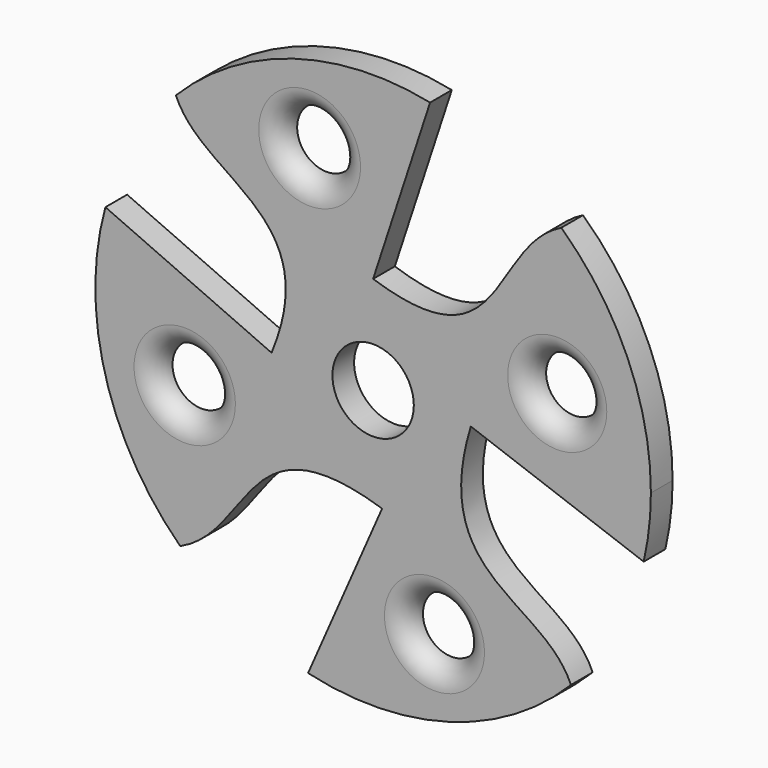
from build123d import *

# Parameters (mm, degrees)
F0_R     = 12.5871716163
F0_R_2   = 12.1953483152
F0_R_3   = 12.6822409032
F0_R_4   = 19.9906816782
F0_R_5   = 12.6370181024
F0_R_6   = 9.5235294205
F0_R_7   = 6.7003849176
F0_R_8   = 6.5953683563
F0_R_9   = 6.9128696082
F0_R_10  = 6.8565575186
F1_DEPTH = 6.35
F2_R     = 5
F4_R     = 5
F6_R     = 5
F8_R     = 5


# Not quite as in the source:
# - a fillet or chamfer that OpenCascade refuses, or shapes differently, is made with other operations: its cross-section is extruded or revolved along the edge and cut away or added


with BuildPart() as f1:
    # F0 (on Front) → F1 (new body)
    with BuildSketch(Plane.XZ):
        with BuildLine():
            ThreePointArc((63.3090875557, -14.7056564815), (64.571840502, -7.4009670899), (64.994591311, 0))
            ThreePointArc((64.994591311, 0), (59.5228001423, 26.1023593361), (44.0287494104, 47.8096865189))
            add(Edge.make_bspline(
                [(44.0287494104, 47.8096865189), (27.5113759255, 39.6058435289), (31.2073216603, 12.5460234383), (0, 22.9526739568)],
                knots=[0, 0, 0, 0, 50.5608726998, 50.5608726998, 50.5608726998, 50.5608726998], degree=3))
            Line((0, 22.9526739568), (13.3303934836, 63.6128721978))
            ThreePointArc((13.3303934836, 63.6128721978), (-18.6797347685, 62.2524249219), (-46.1507096662, 45.7647123556))
            add(Edge.make_bspline(
                [(-46.1507096662, 45.7647123556), (-39.6496795631, 30.4512329053), (-10.8062981221, 31.6188670695), (-23.7553194165, 0)],
                knots=[0, 0, 0, 0, 50.9505878418, 50.9505878418, 50.9505878418, 50.9505878418], degree=3))
            Line((-23.7553194165, 0), (-62.6320905617, 17.3642774556))
            ThreePointArc((-62.6320905617, 17.3642774556), (-62.7024955301, -17.1083007333), (-45.133666011, -46.7680349394))
            add(Edge.make_bspline(
                [(-45.133666011, -46.7680349394), (-28.2305709499, -39.1496551166), (-30.3561454639, -13.2581368089), (2.106344793, -23.6651096493)],
                knots=[0, 0, 0, 0, 52.5867262502, 52.5867262502, 52.5867262502, 52.5867262502], degree=3))
            Line((2.106344793, -23.6651096493), (-15.2139644468, -63.1888612454))
            ThreePointArc((-15.2139644468, -63.1888612454), (17.847761713, -62.4960342863), (46.2891786164, -45.6246516995))
            add(Edge.make_bspline(
                [(46.2891786164, -45.6246516995), (39.8087657789, -30.4243322673), (12.678748928, -33.3952058572), (22.8630993515, 0)],
                knots=[0, 0, 0, 0, 51.2873281857, 51.2873281857, 51.2873281857, 51.2873281857], degree=3))
            Line((22.8630993515, 0), (63.3090875557, -14.7056564815))
        make_face()
        with Locations((-44.0767258406, -13.292982243)):
            Circle(F0_R, mode=Mode.SUBTRACT)
        with Locations((14.3607640639, -45.5371253192)):
            Circle(F0_R_2, mode=Mode.SUBTRACT)
        with Locations((-14.8517312482, 45.0461581349)):
            Circle(F0_R_3, mode=Mode.SUBTRACT)
        Circle(F0_R_4, mode=Mode.SUBTRACT)
        with Locations((43.082293123, 13.3788315579)):
            Circle(F0_R_5, mode=Mode.SUBTRACT)
        Circle(F0_R_4)
        Circle(F0_R_6, mode=Mode.SUBTRACT)
        with Locations((14.3607640639, -45.5371253192)):
            Circle(F0_R_2)
        with Locations((14.3607640639, -45.5371253192)):
            Circle(F0_R_7, mode=Mode.SUBTRACT)
        with Locations((43.082293123, 13.3788315579)):
            Circle(F0_R_5)
        with Locations((43.082293123, 13.3788315579)):
            Circle(F0_R_8, mode=Mode.SUBTRACT)
        with Locations((-14.8517312482, 45.0461581349)):
            Circle(F0_R_3)
        with Locations((-14.8517312482, 45.0461581349)):
            Circle(F0_R_9, mode=Mode.SUBTRACT)
        with Locations((-44.0767258406, -13.292982243)):
            Circle(F0_R)
        with Locations((-44.0767258406, -13.292982243)):
            Circle(F0_R_10, mode=Mode.SUBTRACT)
    extrude(amount=F1_DEPTH)

    # F2
    f2_edges = [f1.edges().sort_by_distance(p)[0] for p in [
        (-21.764601, -6.35, 45.046158),
    ]]
    fillet(f2_edges, radius=F2_R)

    # F3: fillet of radius 5 on 1 edges, made by hand

    # F3_s1 → F3_t2 (revolve, cut)
    with BuildSketch(Plane.XY.offset(45.0461581349)):
        with BuildLine():
            ThreePointArc((-7.93886164, -1.35), (-6.3587432222, -0.3497311906), (-4.5216259151, 0))
            Line((-4.5216259151, 0), (-7.93886164, 0))
            Line((-7.93886164, 0), (-7.93886164, -1.35))
        make_face()
    revolve(axis=Axis((-14.8517312482, 0, 45.0461581349), (0, -1, 0)), mode=Mode.SUBTRACT)

    # F4
    f4_edges = [f1.edges().sort_by_distance(p)[0] for p in [
        (7.660379, -6.35, -45.537125),
    ]]
    fillet(f4_edges, radius=F4_R)

    # F5: fillet of radius 5 on 1 edges, made by hand

    # F5_s1 → F5_t2 (revolve, cut)
    with BuildSketch(Plane.XY.offset(-45.5371253192)):
        with BuildLine():
            ThreePointArc((21.0611489815, -1.35), (22.6412673994, -0.3497311906), (24.4783847065, 0))
            Line((24.4783847065, 0), (21.0611489815, 0))
            Line((21.0611489815, 0), (21.0611489815, -1.35))
        make_face()
    revolve(axis=Axis((14.3607640639, 0, -45.5371253192), (0, -1, 0)), mode=Mode.SUBTRACT)

    # F6
    f6_edges = [f1.edges().sort_by_distance(p)[0] for p in [
        (-50.933283, -6.35, -13.292982),
    ]]
    fillet(f6_edges, radius=F6_R)

    # F7: fillet of radius 5 on 1 edges, made by hand

    # F7_s1 → F7_t2 (revolve, cut)
    with BuildSketch(Plane.XY.offset(-13.292982243)):
        with BuildLine():
            ThreePointArc((-37.220168322, -1.35), (-35.6400499041, -0.3497311906), (-33.802932597, 0))
            Line((-33.802932597, 0), (-37.220168322, 0))
            Line((-37.220168322, 0), (-37.220168322, -1.35))
        make_face()
    revolve(axis=Axis((-44.0767258406, 0, -13.292982243), (0, -1, 0)), mode=Mode.SUBTRACT)

    # F8
    f8_edges = [f1.edges().sort_by_distance(p)[0] for p in [
        (36.486925, -6.35, 13.378832),
    ]]
    fillet(f8_edges, radius=F8_R)

    # F9: fillet of radius 5 on 1 edges, made by hand

    # F9_s1 → F9_t2 (revolve, cut)
    with BuildSketch(Plane.XY.offset(13.3788315579)):
        with BuildLine():
            ThreePointArc((49.6776614793, -1.35), (51.2577798972, -0.3497311906), (53.0948972043, 0))
            Line((53.0948972043, 0), (49.6776614793, 0))
            Line((49.6776614793, 0), (49.6776614793, -1.35))
        make_face()
    revolve(axis=Axis((43.082293123, 0, 13.3788315579), (0, -1, 0)), mode=Mode.SUBTRACT)


solid = f1.part
